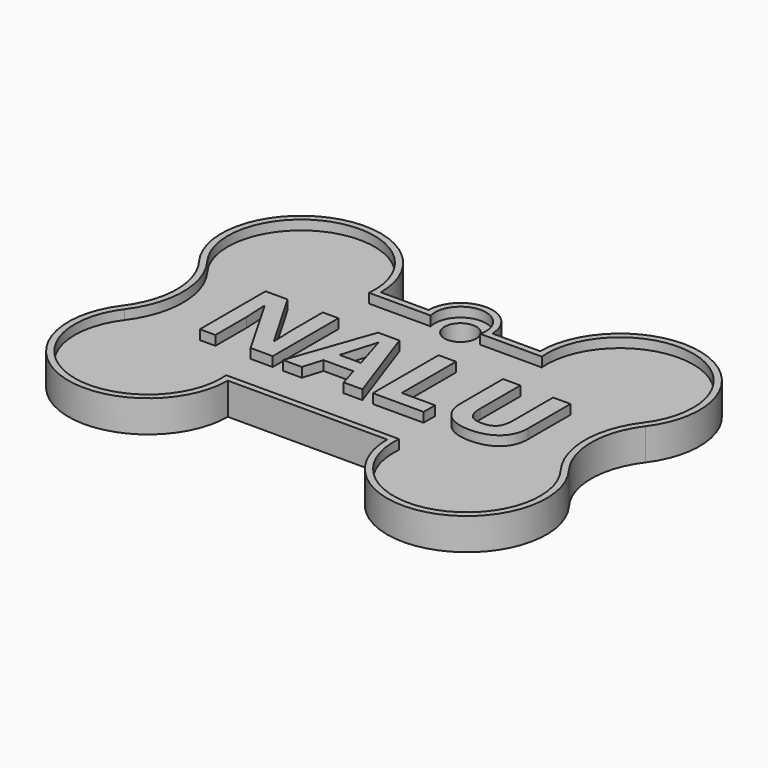
from build123d import *

# Parameters (mm, degrees)
F0_R         = 2.5
F1_DEPTH     = 3.5
F2_TEXT_SIZE = 18.0555555556
F3_DEPTH     = 1.5


# Not quite as in the source:
# - Text() gives the source's letters only with a copy of the font that has no kerning and outlines rounded to 1/6400 em; it was checked with that copy


with BuildPart() as f1:
    # F0 (on Top) → F1 (new body)
    with BuildSketch(Plane.XY):
        with BuildLine():
            ThreePointArc((-10, 7.5), (-3.9528470752, -11.8585412256), (12.5, 0))
            Line((12.5, 0), (37.5, 0))
            ThreePointArc((37.5, 0), (53.9528470752, -11.8585412256), (60, 7.5))
            ThreePointArc((60, 7.5), (57.5, 15), (60, 22.5))
            ThreePointArc((60, 22.5), (53.9528470752, 41.8585412256), (37.5, 30))
            Line((37.5, 30), (30, 30))
            ThreePointArc((30, 30), (25, 35), (20, 30))
            Line((20, 30), (12.5, 30))
            ThreePointArc((12.5, 30), (-3.9528470752, 41.8585412256), (-10, 22.5))
            ThreePointArc((-10, 22.5), (-7.5, 15), (-10, 7.5))
        make_face()
        with Locations((25, 30)):
            Circle(F0_R, mode=Mode.SUBTRACT)
    extrude(amount=F1_DEPTH)

    # F2 (on face) → F3 (join)
    with BuildSketch(Plane.XY.offset(3.5)):
        with BuildLine():
            ThreePointArc((-10, 22.5), (-7.5, 15), (-10, 7.5))
            ThreePointArc((-10, 7.5), (-3.9528470752, -11.8585412256), (12.5, 0))
            Line((12.5, 0), (37.5, 0))
            ThreePointArc((37.5, 0), (53.9528470752, -11.8585412256), (60, 7.5))
            ThreePointArc((60, 7.5), (57.5, 15), (60, 22.5))
            ThreePointArc((60, 22.5), (53.9528470752, 41.8585412256), (37.5, 30))
            Line((37.5, 30), (30, 30))
            ThreePointArc((30, 30), (25, 35), (20, 30))
            Line((20, 30), (12.5, 30))
            ThreePointArc((12.5, 30), (-3.9528470752, 41.8585412256), (-10, 22.5))
        make_face()
        with BuildLine():
            Line((28.8729857316, 29.0000018477), (38.5435587466, 29.0000018477))
            ThreePointArc((38.5435587466, 29.0000018477), (53.1583838963, 41.0577870147), (59.2000014782, 23.0999988914))
            ThreePointArc((59.2000014782, 23.0999988914), (56.5000018477, 15), (59.2000014782, 6.9000011086))
            ThreePointArc((59.2000014782, 6.9000011086), (53.1583838963, -11.0577870147), (38.5435587466, 0.9999981523))
            Line((38.5435587466, 0.9999981523), (11.4564412534, 0.9999981523))
            ThreePointArc((11.4564412534, 0.9999981523), (-3.1583838963, -11.0577870147), (-9.2000014782, 6.9000011086))
            ThreePointArc((-9.2000014782, 6.9000011086), (-6.5000018477, 15), (-9.2000014782, 23.0999988914))
            ThreePointArc((-9.2000014782, 23.0999988914), (-3.1583838963, 41.0577870147), (11.4564412534, 29.0000018477))
            Line((11.4564412534, 29.0000018477), (21.1270142684, 29.0000018477))
            ThreePointArc((21.1270142684, 29.0000018477), (25, 34.0000018477), (28.8729857316, 29.0000018477))
        make_face(mode=Mode.SUBTRACT)
        with Locations((-0.3116319444, 8.5)):
            Text('NALU', F2_TEXT_SIZE, font='Open Sans', font_style=FontStyle.BOLD, text_align=(TextAlign.LEFT, TextAlign.BOTTOM))
    extrude(amount=F3_DEPTH)


solid = f1.part
